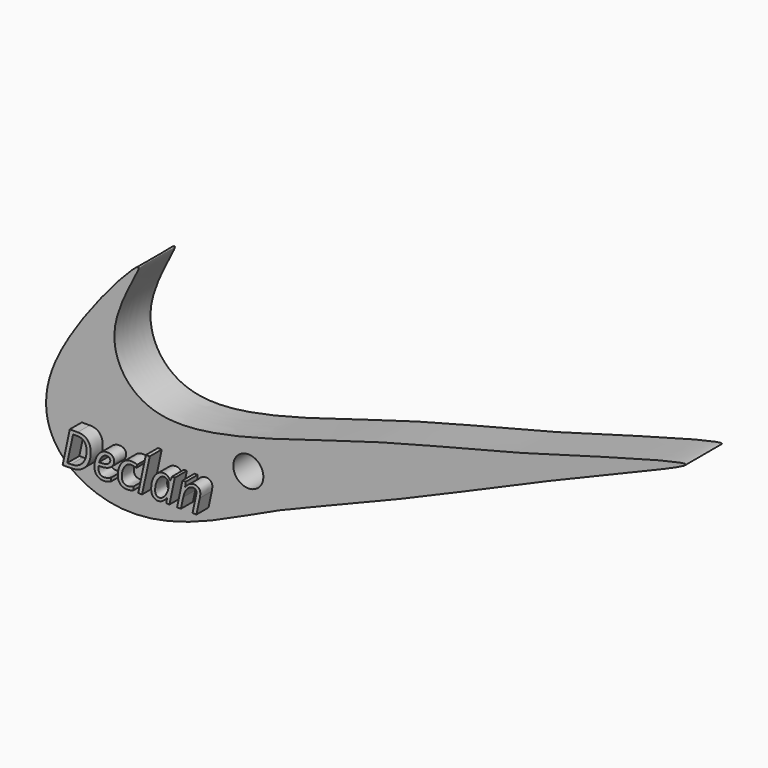
from build123d import *

# Parameters (mm, degrees)
F1_DEPTH     = 6
F2_TEXT_SIZE = 6.3025211501
F3_DEPTH     = 0.8
F4_DEPTH     = 8
F6_D         = 4


# Not quite as in the source:
# - Text() gives the source's letters only with a copy of the font that has no kerning and outlines rounded to 1/6400 em; it was checked with that copy


with BuildPart() as f1:
    # F0 (on Front) → F1 (new body)
    with BuildSketch(Plane.XZ):
        with BuildLine():
            add(Edge.make_bspline(
                [(-77.4006322026, 34.9623523653), (-77.0252452238, 34.8117706714), (-82.7239048963, 26.5862752588), (-77.5842726226, 17.8349116545), (-65.420796951, 18.4388822245), (-47.105884398, 24.7566600449), (-28.4424841641, 29.0604511942), (-16.1253883037, 32.7698671684), (-0.3894311455, 36.9780322845), (-12.9665388691, 31.785743407), (-25.4725422955, 26.6105969392), (-38.5564645752, 20.7668246194), (-50.7887612746, 15.754804622), (-59.7388641462, 12.2871730448), (-68.9650098683, 7.5203834627), (-79.3656946328, 4.7954196344), (-89.2530748908, 9.0023640183), (-91.3811364568, 20.3027984304), (-77.9557237049, 35.1850202343), (-77.4006322026, 34.9623523653)],
                knots=[0, 0, 0, 0, 0.0486962507, 0.0978325361, 0.1533917687, 0.2289959833, 0.3028902738, 0.3683654525, 0.421566038, 0.4675906106, 0.5340447405, 0.5983985672, 0.6596473496, 0.7119872095, 0.7663607377, 0.8213412791, 0.8724327424, 0.927991975, 1, 1, 1, 1], degree=3))
        make_face()
    extrude(amount=F1_DEPTH)

    # F2 (on Front) → F3 (join)
    with BuildSketch(Plane.XZ):
        with Locations((-86.1573591828, 9.8319333047)):
            Text('Declan', F2_TEXT_SIZE, font='Open Sans', font_style=FontStyle.ITALIC, text_align=(TextAlign.LEFT, TextAlign.BOTTOM))
    extrude(amount=F3_DEPTH)

    # F2 (on Front) → F4 (join)
    with BuildSketch(Plane.XZ):
        with Locations((-86.1573591828, 9.8319333047)):
            Text('Declan', F2_TEXT_SIZE, font='Open Sans', font_style=FontStyle.ITALIC, text_align=(TextAlign.LEFT, TextAlign.BOTTOM))
    extrude(amount=F4_DEPTH)

    # F6 (through all)
    with Locations(Plane(origin=(0, 0, 0), x_dir=(1, 0, 0), z_dir=(0, 1, 0))):
        with Locations((-62.7878010273, -15.8038772643)):
            Hole(F6_D / 2)


solid = f1.part
